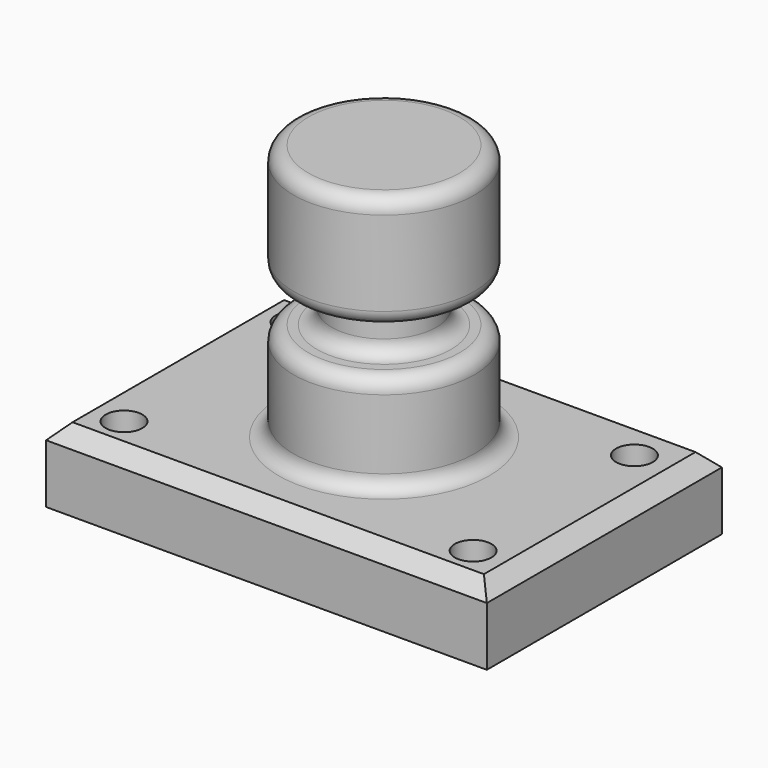
from build123d import *

# Parameters (mm, degrees)
F1_DEPTH = 12.7
F2_R     = 3.175
F3_DEPTH = 25.4
F4_W     = 15.6316435844
F4_H     = 44.45
F6_SIZE  = 2.54
F9_R     = 2.54


# Not quite as in the source:
# - a feature names something its author has since deleted; it is built from what else it names


with BuildPart() as f1:
    # F0 (on Top) → F1 (new body)
    with BuildSketch(Plane.XY):
        Polygon((27.94, 25.4), (-27.94, 25.4), (-38.1, 25.4), (-38.1, 15.24), (-38.1, -15.24), (-38.1, -25.4), (-27.94, -25.4), (27.94, -25.4), (38.1, -25.4), (38.1, -15.24), (38.1, 15.24), (38.1, 25.4), align=None)
    extrude(amount=F1_DEPTH)

    # F2 (on face) → F3 (cut)
    with BuildSketch(Plane.XY.offset(12.7)):
        with Locations((-30.4814037019, 18.666748425)):
            Circle(F2_R)
        with Locations((29.7281444444, 16.9542004048)):
            Circle(F2_R)
        with Locations((30.147915706, -18.4229128063)):
            Circle(F2_R)
        with Locations((-30.2868466824, -18.3251220733)):
            Circle(F2_R)
    extrude(amount=-F3_DEPTH, mode=Mode.SUBTRACT)

    # F4 (on Front) → F5 (revolve)
    with BuildSketch(Plane.XZ):
        with Locations((7.8158217922, 34.925)):
            Rectangle(F4_W, F4_H)
    revolve(axis=Axis((0, 0, 34.925), (0, 0, -1)))

    # F6
    f6_edges = [f1.edges().sort_by_distance(p)[0] for p in [
        (0, -25.4, 12.7),
        (38.1, 0, 12.7),
        (0, 25.4, 12.7),
        (-38.1, 0, 12.7),
    ]]
    chamfer(f6_edges, length=F6_SIZE)

    # F7 (on Front) → F8 (revolve, cut)
    with BuildSketch(Plane.XZ):
        with BuildLine():
            Line((19.2013573515, 37.423838021), (9.0413573515, 37.423838021))
            Line((9.0413573515, 37.423838021), (9.0413573515, 32.343838021))
            ThreePointArc((9.0413573515, 32.343838021), (9.7853061273, 30.5477867968), (11.5813573515, 29.803838021))
            Line((11.5813573515, 29.803838021), (19.2013573515, 29.803838021))
            Line((19.2013573515, 29.803838021), (19.2013573515, 37.423838021))
        make_face()
    revolve(axis=Axis((0, 0, 12.7), (0, 0, 1)), mode=Mode.SUBTRACT)

    # F9
    f9_edges = [f1.edges().sort_by_distance(p)[0] for p in [
        (-15.631644, 0, 12.7),
        (-15.631644, 0, 57.15),
        (15.631644, 0, 21.251919),
        (-15.631644, 0, 29.803838),
        (-15.631644, 0, 37.423838),
        (15.631644, 0, 47.286919),
    ]]
    fillet(f9_edges, radius=F9_R)


solid = f1.part
